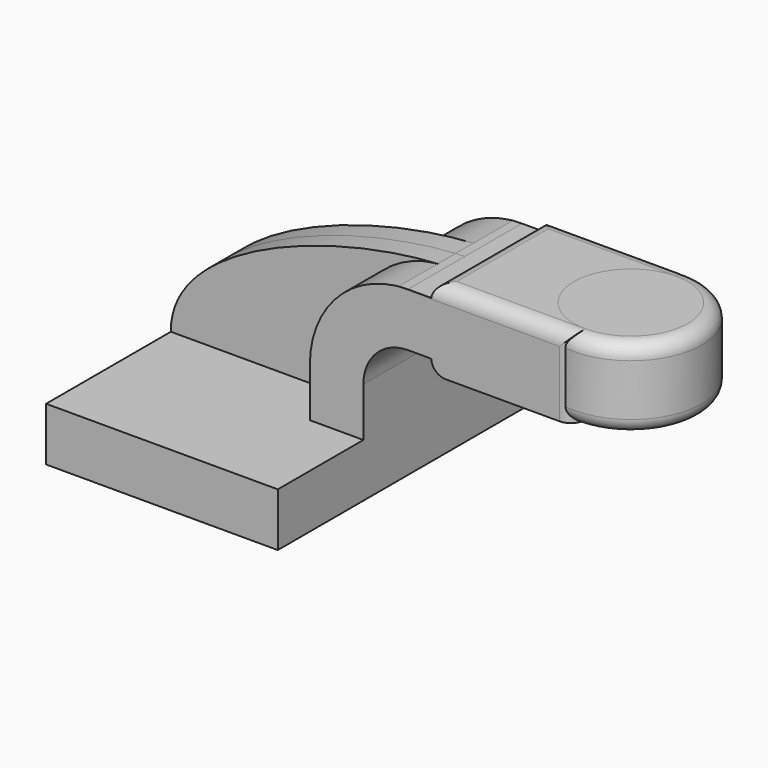
from build123d import *

# Parameters (mm, degrees)
F1_DEPTH    = 63.5
F0_W        = 25.3289441975
F0_H        = 28.575
F2_DEPTH    = 25.4
F3_DEPTH    = 7.9375
F5_T1_DEPTH = 76.2
F5_T3_DEPTH = 76.1542387778
F5_T5_DEPTH = 76.1462857042
F5_T7_DEPTH = 53.975
F5_2_F1_R   = 5.08
F5_2_F2_R   = 5.08


# Not quite as in the source:
# - a fillet or chamfer that OpenCascade refuses, or shapes differently, is made with other operations: its cross-section is extruded or revolved along the edge and cut away or added
# - a feature names something its author has since deleted; it is built from what else it names


with BuildPart() as f1:
    # F0 (on Front) → F1 (new body, symmetric)
    with BuildSketch(Plane.XZ):
        Polygon((-41.275, -9.525), (41.275, -9.525), (41.275, 9.525), (22.225, 9.525), (-41.275, 9.525), align=None)
    extrude(amount=F1_DEPTH, both=True)

    # F0 (on Front) → F2 (join, symmetric)
    with BuildSketch(Plane.XZ):
        with BuildLine():
            Line((22.225, 9.525), (41.275, 9.525))
            Line((41.275, 9.525), (41.275, 27.0002))
            ThreePointArc((41.275, 27.0002), (45.9246798487, 38.2255201513), (57.15, 42.8752))
            Line((57.15, 42.8752), (65.4558, 42.8752))
            Line((65.4558, 42.8752), (65.4558, 61.9252))
            Line((65.4558, 61.9252), (57.15, 61.9252))
            add(Edge.make_bspline(
                [(53.808911529, 61.7650206213), (54.9359515, 61.8330740331), (56.0501940999, 61.8865394151), (57.15, 61.9252)],
                knots=[108.4339478208, 108.4339478208, 108.4339478208, 108.4339478208, 111.5045361635, 111.5045361635, 111.5045361635, 111.5045361635], degree=3))
            ThreePointArc((53.808911529, 61.7650206213), (31.3000179899, 50.484962189), (22.225, 27.0002))
            Line((22.225, 27.0002), (22.225, 9.525))
        make_face()
        Polygon((65.4558, 61.9252), (65.4558, 42.8752), (65.4558, 38.1), (90.9268558025, 38.1), (90.9268558025, 66.675), (65.4558, 66.675), align=None)
        with Locations((103.5913279013, 52.3875)):
            Rectangle(F0_W, F0_H)
    extrude(amount=F2_DEPTH, both=True)

    # F5: fillet of radius 5.08 on 6 edges, made by hand

    # F5_s2 → F5_t1 (cut)
    with BuildSketch(Plane.YZ.offset(52.7558)):
        with BuildLine():
            ThreePointArc((25.4, 61.595), (23.9121024484, 65.1871024484), (20.32, 66.675))
            Line((20.32, 66.675), (25.4, 66.675))
            Line((25.4, 66.675), (25.4, 61.595))
        make_face()
        with BuildLine():
            ThreePointArc((-25.4, 61.595), (-23.9121024484, 65.1871024484), (-20.32, 66.675))
            Line((-20.32, 66.675), (-25.4, 66.675))
            Line((-25.4, 66.675), (-25.4, 61.595))
        make_face()
    extrude(amount=F5_T1_DEPTH, mode=Mode.SUBTRACT)

    # F5_s4 → F5_t3 (cut)
    with BuildSketch(Plane.XZ.offset(-38.0771193889)):
        with BuildLine():
            ThreePointArc((65.4558, 42.8752), (67.0439752185, 39.4817041762), (70.5266477556, 38.1))
            Line((70.5266477556, 38.1), (65.4558, 38.1))
            Line((65.4558, 38.1), (65.4558, 42.8752))
        make_face()
    extrude(amount=F5_T3_DEPTH, mode=Mode.SUBTRACT)

    # F5_s6 → F5_t5 (cut)
    with BuildSketch(Plane.XZ.offset(-38.0731428521)):
        with BuildLine():
            ThreePointArc((70.5250571408, 66.675), (67.0516593807, 65.3020079579), (65.4558, 61.9252))
            Line((65.4558, 61.9252), (65.4558, 66.675))
            Line((65.4558, 66.675), (70.5250571408, 66.675))
        make_face()
    extrude(amount=F5_T5_DEPTH, mode=Mode.SUBTRACT)

    # F5_s8 → F5_t7 (cut)
    with BuildSketch(Plane.XY.offset(25.4)):
        with BuildLine():
            ThreePointArc((111.1758, -25.4), (114.7679024484, -23.9121024484), (116.2558, -20.32))
            Line((116.2558, -20.32), (116.2558, -25.4))
            Line((116.2558, -25.4), (111.1758, -25.4))
        make_face()
        with BuildLine():
            ThreePointArc((111.1758, 25.4), (114.7679024484, 23.9121024484), (116.2558, 20.32))
            Line((116.2558, 20.32), (116.2558, 25.4))
            Line((116.2558, 25.4), (111.1758, 25.4))
        make_face()
    extrude(amount=F5_T7_DEPTH, mode=Mode.SUBTRACT)


with BuildPart() as f3:
    # F0 (on Front) → F3 (new body, symmetric)
    with BuildSketch(Plane.XZ):
        with BuildLine():
            add(Edge.make_bspline(
                [(-41.275, 9.525), (-41.7501631131, 38.7664319524), (14.0089189004, 59.3618003655), (53.808911529, 61.7650206213)],
                knots=[0, 0, 0, 0, 108.4339478208, 108.4339478208, 108.4339478208, 108.4339478208], degree=3))
            Line((-41.275, 9.525), (22.225, 9.525))
            Line((22.225, 9.525), (22.225, 27.0002))
            ThreePointArc((22.225, 27.0002), (31.3000179899, 50.484962189), (53.808911529, 61.7650206213))
        make_face()
    extrude(amount=F3_DEPTH, both=True)


with BuildPart() as f4:
    # F0 (on Front) → F4 (revolve)
    with BuildSketch(Plane.XZ):
        with Locations((103.5913279013, 52.3875)):
            Rectangle(F0_W, F0_H)
    revolve(axis=Axis((116.2558, 0, 52.3875), (0, 0, 1)))

    # F5#2: fillet of radius 5.08 on 2 edges, made by hand

    # F5_2_f1
    f5_2_f1_edges = [f4.edges().sort_by_distance(p)[0] for p in [
        (141.5847441975, 0, 66.675),
    ]]
    fillet(f5_2_f1_edges, radius=F5_2_F1_R)

    # F5_2_f2
    f5_2_f2_edges = [f4.edges().sort_by_distance(p)[0] for p in [
        (141.5847441975, 0, 38.1),
    ]]
    fillet(f5_2_f2_edges, radius=F5_2_F2_R)


solid = Compound([f1.part, f3.part, f4.part])
